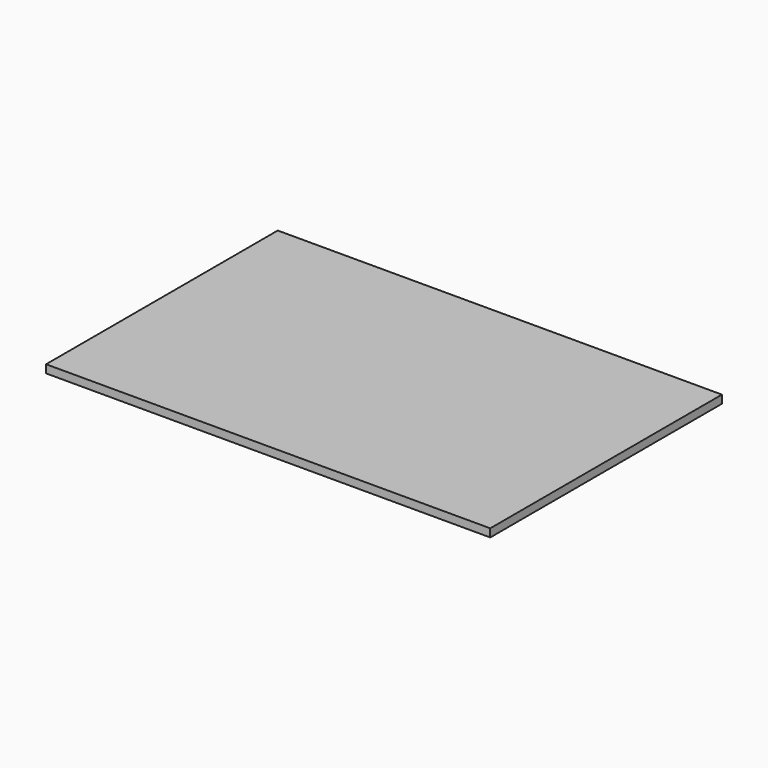
from build123d import *

# Parameters (mm, degrees)
F10_W     = 879.9634585157
F10_H     = 573.7158786505
F11_DEPTH = 6
F12_DEPTH = 10


# Not quite as in the source:
# - a feature of the source that left no trace in its solid (it failed there, or was rolled back) is left out


with BuildPart() as f11:
    # F10 (on face) → F11 (new body)
    with BuildSketch(Plane.XY.offset(380)):
        with Locations((449.9826724641, 269.9618572369)):
            Rectangle(F10_W, F10_H)
    extrude(amount=-F11_DEPTH)

    # F12 (add): a face of the model
    f12_faces = [f11.faces().sort_by_distance(p)[0] for p in [
        (449.9826724641, 269.9618572369, 380),
    ]]
    extrude(f12_faces, amount=F12_DEPTH)


solid = f11.part
